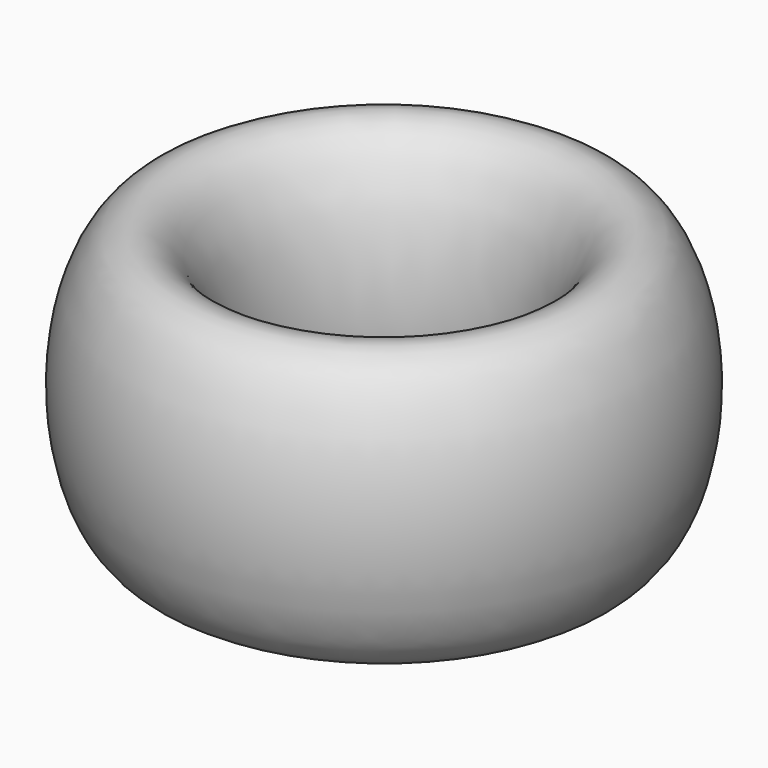
from build123d import *


with BuildPart() as f2:
    # F0 (on Front) → F2 (revolve)
    with BuildSketch(Plane.XZ):
        with BuildLine():
            Line((0, 43.5657091439), (0, -43.5657091439))
            add(Edge.make_bspline(
                [(0, -43.5657091439), (20.9509272428, -43.5657091439), (20.9509272428, 0), (20.9509272428, 43.5657091439), (0, 43.5657091439)],
                knots=[0, 0, 0, 1.5707963268, 1.5707963268, 3.1415926536, 3.1415926536, 3.1415926536], degree=2, weights=[1, 0.7071067812, 1, 0.7071067812, 1]))
        make_face()
        with BuildLine():
            add(Edge.make_bspline(
                [(0, 43.5657091439), (-20.9509272428, 43.5657091439), (-20.9509272428, 0), (-20.9509272428, -43.5657091439), (0, -43.5657091439)],
                knots=[3.1415926536, 3.1415926536, 3.1415926536, 4.7123889804, 4.7123889804, 6.2831853072, 6.2831853072, 6.2831853072], degree=2, weights=[1, 0.7071067812, 1, 0.7071067812, 1]))
            Line((0, -43.5657091439), (0, 43.5657091439))
        make_face()
    revolve(axis=Axis((-61.5957416594, 0, -2.6460923254), (0, 0, -1)))


solid = f2.part
